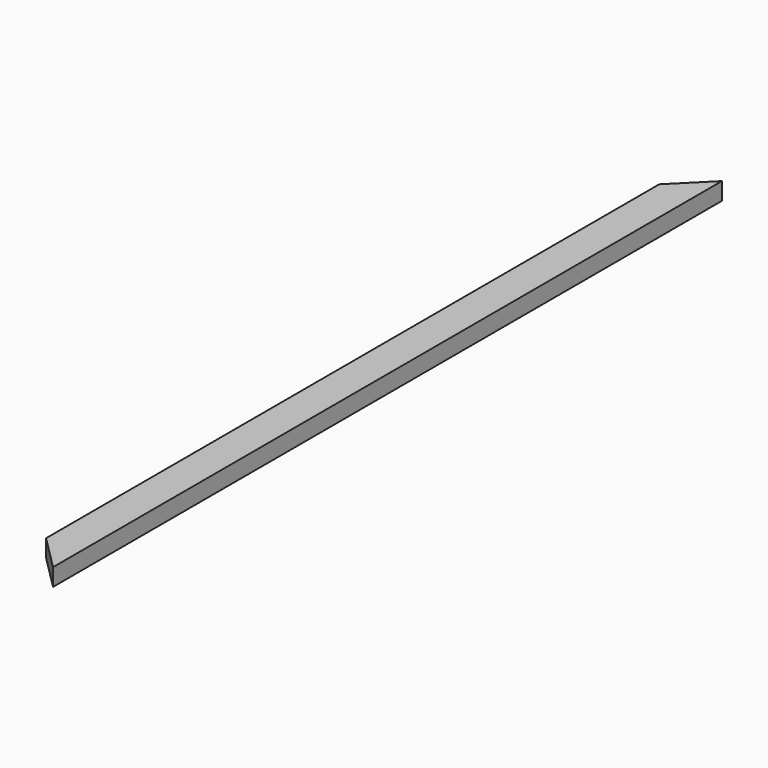
from build123d import *

# Parameters (mm, degrees)
F0_W     = 50.8
F0_H     = 25.4
F1_DEPTH = 1219.2
F2_SIZE  = 50.79999
F3_SIZE  = 50.79999


# Not quite as in the source:
# - a fillet or chamfer is up to 0.001 mm smaller than in the source, because OpenCascade refuses the exact size


with BuildPart() as f1:
    # F0 (on Front) → F1 (new body)
    with BuildSketch(Plane.XZ):
        with Locations((-39.6967977285, 43.9715571764)):
            Rectangle(F0_W, F0_H)
    extrude(amount=F1_DEPTH)

    # F2 (size 50.8 in the source; OpenCascade refuses exactly that, so slightly less here)
    f2_edges = [f1.edges().sort_by_distance(p)[0] for p in [
        (-65.096798, 0, 43.971557),
    ]]
    chamfer(f2_edges, length=F2_SIZE)

    # F3 (size 50.8 in the source; OpenCascade refuses exactly that, so slightly less here)
    f3_edges = [f1.edges().sort_by_distance(p)[0] for p in [
        (-65.096798, -1219.2, 43.971557),
    ]]
    chamfer(f3_edges, length=F3_SIZE)


solid = f1.part
